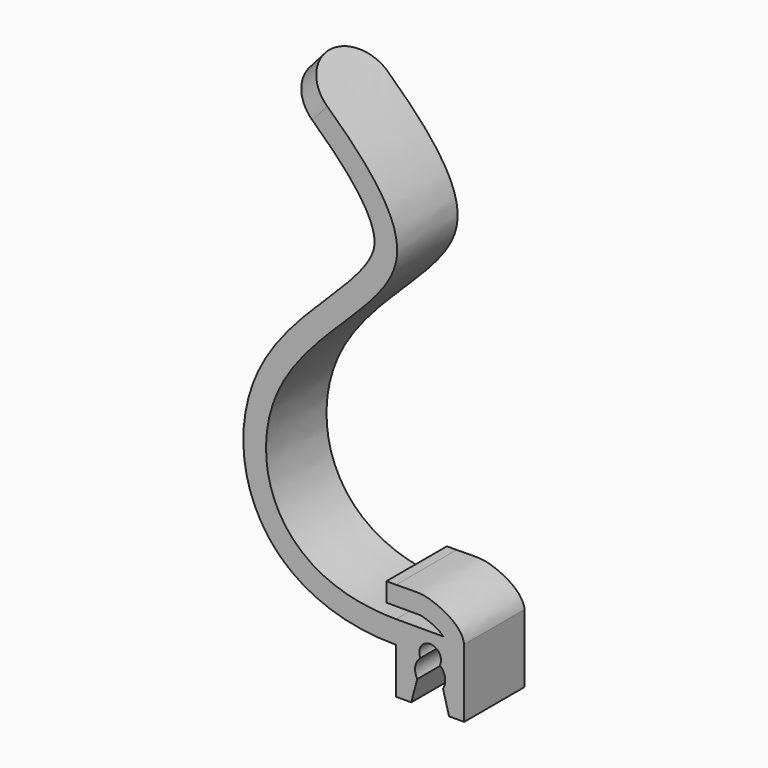
from build123d import *

# Parameters (mm, degrees)
F0_W     = 1.2820525234
F0_H     = 2.5
F1_DEPTH = 10
F2_R     = 4.99999


# Not quite as in the source:
# - a fillet or chamfer is up to 0.001 mm smaller than in the source, because OpenCascade refuses the exact size
# - ends of sketch curves that miss each other by under 0.0002 mm in the source are joined
# - the dataset's text gives a spline's control points without its knots; the knots are read off the source's solid


with BuildPart() as f1:
    # F0 (on Front) → F1 (new body)
    with BuildSketch(Plane.XZ):
        with BuildLine():
            add(Edge.make_bspline(
                [(-12.8351654857, 60.0928552449), (-5.7875354147, 53.906599191), (8.777936679, 40.5694219601), (-23.1086700941, 24.0621289914), (-16.0203649173, 0), (0, 0)],
                knots=[0, 0, 0, 0, 0.3165523806, 0.6579654054, 1, 1, 1, 1], degree=3))
            Line((-12.8351654857, 60.0928552449), (-14.8142245089, 57.8382321316))
            add(Edge.make_bspline(
                [(-14.8142245089, 57.8382321316), (-13.4290580966, 56.6223632484), (-10.691125206, 54.1981610075), (-7.6731453742, 51.234903206), (-5.7031473114, 48.9646975714), (-4.4973442137, 47.3389761791), (-3.6065055701, 45.8268027586), (-3.0562892839, 44.4767256425), (-2.8691798622, 43.5244251506), (-2.8533853893, 42.8539466076), (-2.894828603, 42.4583864203), (-2.9591120331, 42.1477668912), (-3.050219873, 41.8177440392), (-3.2183868875, 41.3682546958), (-3.5175315945, 40.768166554), (-4.0504649627, 39.8959215446), (-4.9630892195, 38.6909645325), (-6.3905967255, 37.1116155569), (-8.066687543, 35.420116471), (-10.5198350501, 33.0160284917), (-13.1348534089, 30.3688644412), (-15.5842649886, 27.3797874151), (-16.9735136512, 25.3382900326), (-17.9499152533, 23.5844597655), (-18.6017035016, 22.2031022914), (-19.1536832643, 20.7619148102), (-19.7416120825, 18.7948578312), (-20.19708073, 16.2597361699), (-20.2646454432, 13.1608601555), (-19.813608931, 10.0714160991), (-18.7972924536, 7.0717848528), (-17.1727615016, 4.2632836685), (-14.9191394115, 1.7675069189), (-12.0511132397, -0.2942248007), (-8.6069967787, -1.8291372046), (-4.6185416475, -2.7802993331), (-1.6010535304, -3), (0, -3)],
                knots=[0, 0, 0, 0, 0.0625, 0.125, 0.15625, 0.1875, 0.21875, 0.25, 0.28125, 0.296875, 0.3125, 0.3203125, 0.328125, 0.34375, 0.359375, 0.375, 0.40625, 0.4375, 0.46875, 0.5, 0.5625, 0.59375, 0.625, 0.640625, 0.65625, 0.671875, 0.6875, 0.71875, 0.75, 0.78125, 0.8125, 0.84375, 0.875, 0.90625, 0.9375, 0.96875, 1, 1, 1, 1], degree=3))
            Line((0, -3), (0, -9.0464234526))
            Line((0, -9.0464234526), (2, -9.0464234526))
            Line((2, -9.0464234526), (2.7974422544, -6.0703284432))
            ThreePointArc((2.7974422544, -6.0703284432), (2.5255002285, -4.7025452259), (3.213551795, -3.489545458))
            ThreePointArc((3.213551795, -3.489545458), (4.5, -1.4279751142), (5.786448205, -3.489545458))
            ThreePointArc((5.786448205, -3.489545458), (6.4744997715, -4.7025452259), (6.2025577456, -6.0703284432))
            Line((6.2025577456, -6.0703284432), (7, -9.0464234526))
            Line((7, -9.0464234526), (9, -9.0464234526))
            Line((9, -9.0464234526), (9, 0))
            Line((9, 0), (6.2733793459, 0))
            Line((6.2733793459, 0), (0, 0))
        make_face()
        with BuildLine():
            add(Edge.make_bspline(
                [(6.2733793459, -2.59666e-05), (6.2592824776, 0.014416612), (6.1587188988, 0.1147915999), (5.9165734192, 0.3206018905), (5.4806109561, 0.6104131264), (4.9836673607, 0.8790221572), (4.4683758095, 1.1099751491), (4.0613635378, 1.2618551318), (3.7711795239, 1.3558647219), (3.5221420098, 1.4279920473), (3.3221876047, 1.472810754), (3.1905104971, 1.4932113257), (3.1342551744, 1.5000753278)],
                knots=[0.176762631, 0.176762631, 0.176762631, 0.176762631, 0.1875, 0.25, 0.3125, 0.375, 0.4375, 0.5, 0.53125, 0.5625, 0.625, 0.6684456144, 0.6684456144, 0.6684456144, 0.6684456144], degree=3))
            Line((6.2733793459, -2.59666e-05), (9, 0))
            add(Edge.make_bspline(
                [(9, 0), (8.7126399678, 2.0028417389), (3.7508158887, 4.3720863792), (2.5718559585, 3.9896494504), (0, 4)],
                knots=[0, 0, 0, 0, 0.5326615286, 1, 1, 1, 1], degree=3))
            Line((0, 4), (0, 1.5))
            Line((0, 1.5), (3.1342551744, 1.5000753278))
        make_face()
        with Locations((-0.6410262617, 2.75)):
            Rectangle(F0_W, F0_H)
    extrude(amount=F1_DEPTH)

    # F2 (radius 5 in the source; OpenCascade refuses exactly that, so slightly less here)
    f2_edges = [f1.edges().sort_by_distance(p)[0] for p in [
        (-13.824695, -10, 58.965544),
        (-13.824695, 0, 58.965544),
    ]]
    fillet(f2_edges, radius=F2_R)


solid = f1.part
